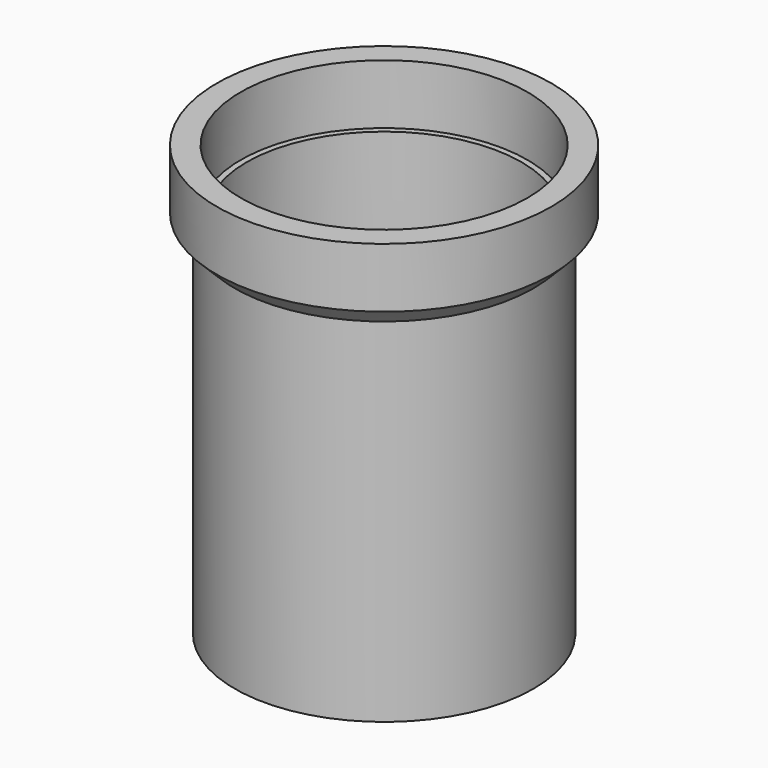
from build123d import *

# Parameters (mm, degrees)
F0_R     = 25
F0_R_2   = 5
F1_DEPTH = 45
F2_SIZE2 = 17
F2_SIZE  = 12.5
F3_R     = 25
F3_R_2   = 23
F4_DEPTH = 17
F5_R     = 28
F5_R_2   = 25
F5_R_3   = 24
F6_DEPTH = 10
F7_SIZE  = 2.99999
F8_SIZE2 = 30
F8_SIZE  = 5


# Not quite as in the source:
# - a fillet or chamfer is up to 0.001 mm smaller than in the source, because OpenCascade refuses the exact size


with BuildPart() as f1:
    # F0 (on Top) → F1 (new body)
    with BuildSketch(Plane.XY):
        Circle(F0_R)
        Circle(F0_R_2, mode=Mode.SUBTRACT)
    extrude(amount=F1_DEPTH)

    # F2
    f2_edges = [f1.edges().sort_by_distance(p)[0] for p in [
        (-5, 0, 45),
    ]]
    f2_side = f1.faces().sort_by_distance((-5, 0, 22.5))[0]
    chamfer(f2_edges, length=F2_SIZE, length2=F2_SIZE2, reference=f2_side)

    # F3 (on face) → F4 (join)
    with BuildSketch(Plane.XY.offset(45)):
        Circle(F3_R)
        Circle(F3_R_2, mode=Mode.SUBTRACT)
    extrude(amount=F4_DEPTH)

    # F5 (on face) → F6 (join)
    with BuildSketch(Plane.XY.offset(62)):
        Circle(F5_R)
        Circle(F5_R_2, mode=Mode.SUBTRACT)
        Circle(F5_R_2)
        Circle(F5_R_3, mode=Mode.SUBTRACT)
    extrude(amount=F6_DEPTH)

    # F7 (size 3 in the source; OpenCascade refuses exactly that, so slightly less here)
    f7_edges = [f1.edges().sort_by_distance(p)[0] for p in [
        (-25, 0, 62),
    ]]
    chamfer(f7_edges, length=F7_SIZE)

    # F8
    f8_edges = [f1.edges().sort_by_distance(p)[0] for p in [
        (-5, 0, 0),
    ]]
    f8_side = f1.faces().sort_by_distance((-24.292893, 0, 0))[0]
    chamfer(f8_edges, length=F8_SIZE, length2=F8_SIZE2, reference=f8_side)


solid = f1.part
